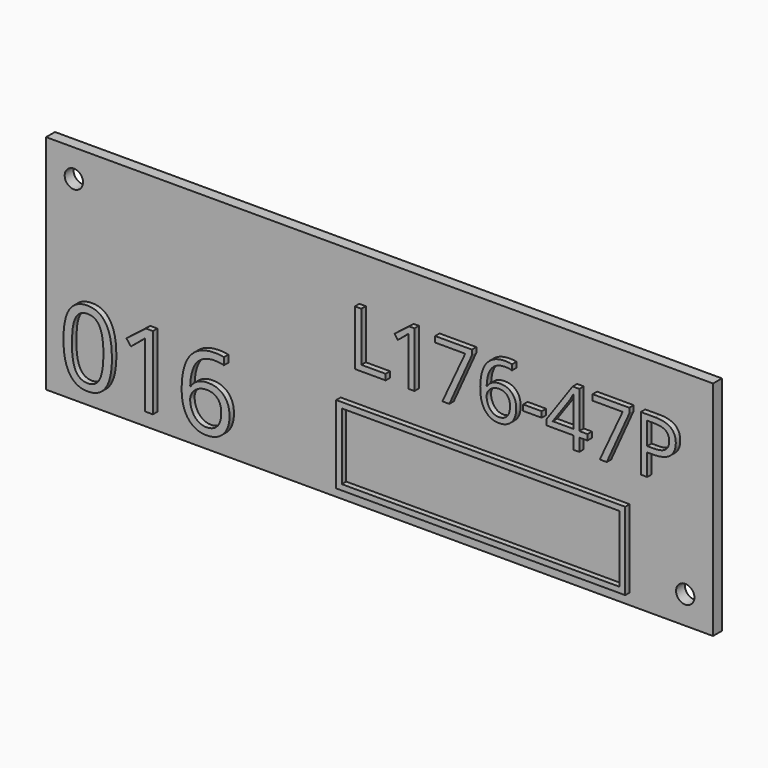
from build123d import *

# Parameters (mm, degrees)
F0_W         = 120
F0_H         = 40
F1_DEPTH     = 2
F3_D         = 3.3
F4_TEXT_SIZE = 13.9049826188
F5_DEPTH     = 1
F6_TEXT_SIZE = 18.4837545126
F7_DEPTH     = 1
F8_W         = 52
F8_H         = 14
F8_W_2       = 49.99999962
F8_H_2       = 11.99999962
F9_DEPTH     = 1


# Not quite as in the source:
# - Text() gives the source's letters only with a copy of the font that has no kerning and outlines rounded to 1/6400 em; it was checked with that copy


with BuildPart() as f1:
    # F0 (on Front) → F1 (new body)
    with BuildSketch(Plane.XZ):
        Rectangle(F0_W, F0_H)
    extrude(amount=F1_DEPTH)

    # F3 (through all)
    with Locations(Plane.XZ.offset(2)):
        with Locations((-55, 15), (55, -15)):
            Hole(F3_D / 2)

    # F4 (on face) → F5 (join)
    with BuildSketch(Plane.XZ.offset(2)):
        with Locations((-5, 2)):
            Text('L176-47P', F4_TEXT_SIZE, font='Open Sans', text_align=(TextAlign.LEFT, TextAlign.BOTTOM))
    extrude(amount=F5_DEPTH)

    # F6 (on face) → F7 (join)
    with BuildSketch(Plane.XZ.offset(2)):
        with Locations((-57, -17)):
            Text('016', F6_TEXT_SIZE, font='Open Sans', text_align=(TextAlign.LEFT, TextAlign.BOTTOM))
    extrude(amount=F7_DEPTH)

    # F8 (on face) → F9 (join)
    with BuildSketch(Plane.XZ.offset(2)):
        with Locations((19, -11)):
            Rectangle(F8_W, F8_H)
        with Locations((19, -11)):
            Rectangle(F8_W_2, F8_H_2, mode=Mode.SUBTRACT)
    extrude(amount=F9_DEPTH)


solid = f1.part
